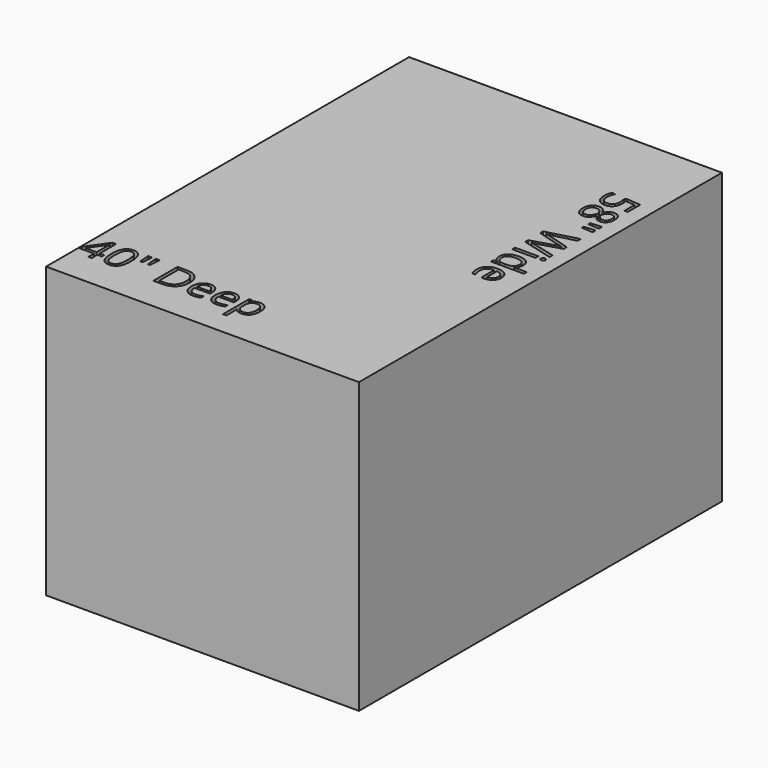
from build123d import *

# Parameters (mm, degrees)
F0_W           = 1016
F0_H           = 1473.2
F1_DEPTH       = 939.8
F2_TEXT_SIZE   = 141.1111111111
F2_TEXT_SIZE_2 = 137.2890339957
F3_DEPTH       = 25.4


# Not quite as in the source:
# - Text() gives the source's letters only with a copy of the font that has no kerning and outlines rounded to 1/6400 em; it was checked with that copy


with BuildPart() as f1:
    # F0 (on Top) → F1 (new body)
    with BuildSketch(Plane.XY):
        with Locations((0, 127)):
            Rectangle(F0_W, F0_H)
    extrude(amount=F1_DEPTH)

    # F2 (on face) → F3 (cut)
    with BuildSketch(Plane.XY.offset(939.8)):
        with Locations(Location((355.6, 611.7843460174), (0, 0, -90))):
            Text('58" Wide', F2_TEXT_SIZE, font='Open Sans', text_align=(TextAlign.LEFT, TextAlign.BOTTOM))
        with Locations((-508, -500.6133317947)):
            Text('40" Deep', F2_TEXT_SIZE_2, font='Open Sans', text_align=(TextAlign.LEFT, TextAlign.BOTTOM))
    extrude(amount=-F3_DEPTH, mode=Mode.SUBTRACT)


solid = f1.part
